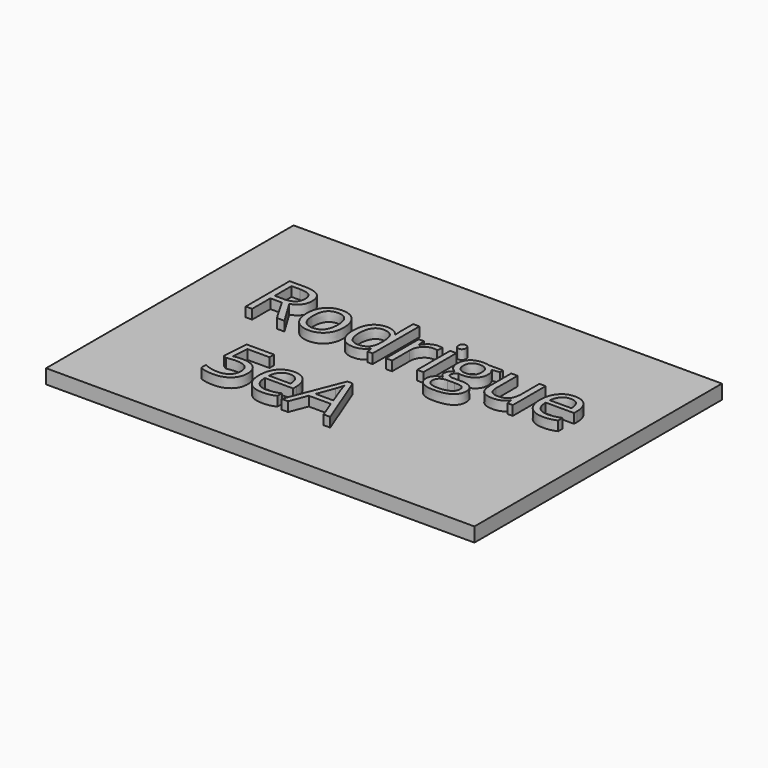
from build123d import *

# Parameters (mm, degrees)
F0_W         = 90
F0_H         = 65
F1_DEPTH     = 3
F2_TEXT_SIZE = 16.1494361237
F3_DEPTH     = 2
F4_DEPTH     = 2


# Not quite as in the source:
# - Text() gives the source's letters only with a copy of the font that has no kerning and outlines rounded to 1/6400 em; it was checked with that copy


with BuildPart() as f1:
    # F0 (on Top) → F1 (new body)
    with BuildSketch(Plane.XY):
        with Locations((45, -32.5)):
            Rectangle(F0_W, F0_H)
    extrude(amount=F1_DEPTH)

    # F2 (on face) → F3 (join)
    with BuildSketch(Plane.XY.offset(3)):
        with Locations((12.6974936575, -30.4127056152)):
            Text('Rodrigue', F2_TEXT_SIZE, font='Open Sans', text_align=(TextAlign.LEFT, TextAlign.BOTTOM))
        with Locations((21.090153743, -52.3759387434)):
            Text('5eA', F2_TEXT_SIZE, font='Open Sans', text_align=(TextAlign.LEFT, TextAlign.BOTTOM))
    extrude(amount=F3_DEPTH)

    # F2 (on face) → F4 (join)
    with BuildSketch(Plane.XY.offset(3)):
        with Locations((12.6974936575, -30.4127056152)):
            Text('Rodrigue', F2_TEXT_SIZE, font='Open Sans', text_align=(TextAlign.LEFT, TextAlign.BOTTOM))
        with Locations((21.090153743, -52.3759387434)):
            Text('5eA', F2_TEXT_SIZE, font='Open Sans', text_align=(TextAlign.LEFT, TextAlign.BOTTOM))
    extrude(amount=F4_DEPTH)


solid = f1.part
